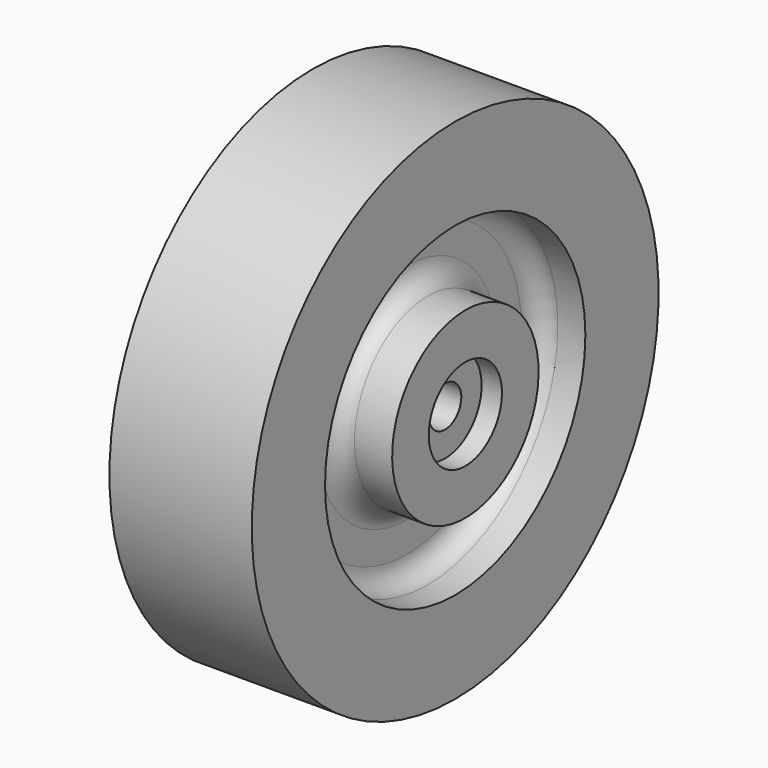
from build123d import *

# Parameters (mm, degrees)
F2_R        = 7.14375
F2_R_2      = 3.175
F3_DEPTH    = 22.225
F1_FACE_R   = 14.2875
F1_FACE_R_2 = 7.14375
F3_FACE_R   = 7.14375
F3_FACE_R_2 = 3.175
F4_DEPTH    = 3.175


with BuildPart() as f1:
    # F0 (on Front) → F1 (revolve)
    with BuildSketch(Plane.XZ):
        with BuildLine():
            Line((-12.7, 0), (0, 0))
            Line((0, 0), (0, 32.54375))
            Line((0, 32.54375), (-11.1125, 32.54375))
            Line((-11.1125, 32.54375), (-11.1125, 18.25625))
            Line((-11.1125, 18.25625), (-6.8100053257, 18.25625))
            ThreePointArc((-6.8100053257, 18.25625), (-4.5649412955, 17.3263140303), (-3.6350053257, 15.08125))
            Line((-3.6350053257, 15.08125), (-3.6350053257, 10.31875))
            ThreePointArc((-3.6350053257, 10.31875), (-4.5649412955, 8.0736859697), (-6.8100053257, 7.14375))
            Line((-6.8100053257, 7.14375), (-12.7, 7.14375))
            Line((-12.7, 7.14375), (-12.7, 0))
        make_face()
        with BuildLine():
            Line((0, 32.54375), (0, 0))
            Line((0, 0), (12.7, 0))
            Line((12.7, 0), (12.7, 7.14375))
            Line((12.7, 7.14375), (6.8100053257, 7.14375))
            ThreePointArc((6.8100053257, 7.14375), (4.5649412955, 8.0736859697), (3.6350053257, 10.31875))
            Line((3.6350053257, 10.31875), (3.6350053257, 15.08125))
            ThreePointArc((3.6350053257, 15.08125), (4.5649412955, 17.3263140303), (6.8100053257, 18.25625))
            Line((6.8100053257, 18.25625), (11.1125, 18.25625))
            Line((11.1125, 18.25625), (11.1125, 32.54375))
            Line((11.1125, 32.54375), (0, 32.54375))
        make_face()
    revolve(axis=Axis((-12.7447592095, 0, -7.14375), (-1, 0, 0)))


with BuildPart() as f3:
    # F2 (on face) → F3 (new body)
    with BuildSketch(Plane(origin=(-12.7, 0, 0), x_dir=(0, -1, 0), z_dir=(-1, 0, 0))):
        with Locations((0, -7.14375)):
            Circle(F2_R)
        with Locations((0, -7.14375)):
            Circle(F2_R_2, mode=Mode.SUBTRACT)
    extrude(amount=-F3_DEPTH)

    # F1_face (on face) + F3_face (on face) → F4 (join)
    with BuildSketch(Plane(origin=(-12.7, 0, -7.14375), x_dir=(0, -1, 0), z_dir=(-1, 0, 0))):
        Circle(F1_FACE_R)
        Circle(F1_FACE_R_2, mode=Mode.SUBTRACT)
    with BuildSketch(Plane(origin=(-12.7, 0, -7.14375), x_dir=(0, -1, 0), z_dir=(-1, 0, 0))):
        Circle(F3_FACE_R)
        Circle(F3_FACE_R_2, mode=Mode.SUBTRACT)
    extrude(amount=F4_DEPTH)


solid = Compound([f1.part, f3.part])
